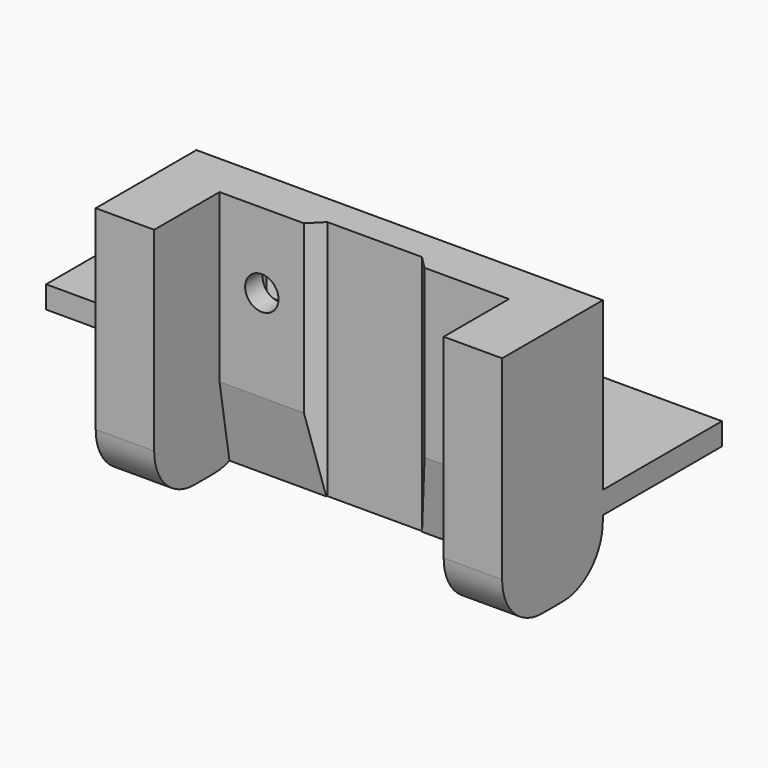
from build123d import *

# Parameters (mm, degrees)
F0_W           = 13.375
F0_H           = 2
F1_DEPTH       = 25
F2_R           = 1.75
F3_DEPTH       = 2
F4_W           = 11.3
F4_H           = 7
F5_DEPTH       = 25
F5_DEPTH_BACK  = 11.5
F6_W           = 26
F6_H           = 6.5
F7_DEPTH       = 7
F9_DEPTH       = 7
F11_DEPTH      = 19.75
F11_DEPTH_BACK = 6.25
F12_T1_DEPTH   = 27.75
F12_T3_DEPTH   = 27.75
F12_T5_DEPTH   = 59
F14_DEPTH      = 15
F15_W          = 5.5
F15_H          = 5.5
F16_DEPTH      = 2
F17_DEPTH      = 2
F18_D          = 3


# Not quite as in the source:
# - a fillet or chamfer that OpenCascade refuses, or shapes differently, is made with other operations: its cross-section is extruded or revolved along the edge and cut away or added


with BuildPart() as f1:
    # F0 (on Right) → F1 (new body, symmetric)
    with BuildSketch(Plane.YZ):
        with Locations((6.6875, 1)):
            Rectangle(F0_W, F0_H)
    extrude(amount=F1_DEPTH, both=True)

    # F2 (on face) → F3 (cut, through all)
    with BuildSketch(Plane.XY.offset(2)):
        with Locations((-13, 4)):
            Circle(F2_R)
        with Locations((13, 4)):
            Circle(F2_R)
    extrude(amount=-F3_DEPTH, mode=Mode.SUBTRACT)

    # F4 (on Right) → F5 (join, two sides)
    with BuildSketch(Plane.YZ) as f5_sk:
        with Locations((-5.65, -1.5)):
            Rectangle(F4_W, F4_H)
    extrude(amount=F5_DEPTH)
    extrude(f5_sk.sketch, amount=-F5_DEPTH_BACK)

    # F6 (on face) → F7 (cut, through all)
    with BuildSketch(Plane(origin=(0, 0, -5), x_dir=(1, 0, 0), z_dir=(0, 0, -1))):
        with Locations((6.75, 8.05)):
            Rectangle(F6_W, F6_H)
    extrude(amount=-F7_DEPTH, mode=Mode.SUBTRACT)

    # F8 (on face) → F9 (cut, through all)
    with BuildSketch(Plane(origin=(0, 0, -5), x_dir=(1, 0, 0), z_dir=(0, 0, -1))):
        Polygon((13, 4.8), (0.5, 4.8), (2.5, 2.8), (11, 2.8), align=None)
    extrude(amount=-F9_DEPTH, mode=Mode.SUBTRACT)

    # F10 (on Right) → F11 (cut, two sides)
    with BuildSketch(Plane.YZ) as f11_sk:
        Polygon((-4.8, -5), (-2.8, -5), (-4.8, 7), align=None)
    extrude(amount=F11_DEPTH, mode=Mode.SUBTRACT)
    extrude(f11_sk.sketch, amount=-F11_DEPTH_BACK, mode=Mode.SUBTRACT)

    # F12: fillet of radius 4.5 on 3 edges, made by hand

    # F12_s2 → F12_t1 (cut)
    with BuildSketch(Plane.YZ.offset(-22.75)):
        with BuildLine():
            ThreePointArc((-6.8, -5), (-9.9819805153, -3.6819805153), (-11.3, -0.5))
            Line((-11.3, -0.5), (-11.3, -5))
            Line((-11.3, -5), (-6.8, -5))
        make_face()
    extrude(amount=F12_T1_DEPTH, mode=Mode.SUBTRACT)

    # F12_s4 → F12_t3 (cut)
    with BuildSketch(Plane.YZ.offset(8.5)):
        with BuildLine():
            ThreePointArc((-6.8, -5), (-9.9819805153, -3.6819805153), (-11.3, -0.5))
            Line((-11.3, -0.5), (-11.3, -5))
            Line((-11.3, -5), (-6.8, -5))
        make_face()
    extrude(amount=F12_T3_DEPTH, mode=Mode.SUBTRACT)

    # F12_s6 → F12_t5 (cut)
    with BuildSketch(Plane.YZ.offset(-22.75)):
        with BuildLine():
            ThreePointArc((0, -0.5), (-1.3180194847, -3.6819805153), (-4.5, -5))
            Line((-4.5, -5), (0, -5))
            Line((0, -5), (0, -0.5))
        make_face()
    extrude(amount=F12_T5_DEPTH, mode=Mode.SUBTRACT)

    # F13 (on face) → F14 (join)
    with BuildSketch(Plane.XY.offset(2)):
        Polygon((25, 0), (-11.5, 0), (-11.5, -11.3), (-6.25, -11.3), (-6.25, -3.9666666667), (1.3333333333, -3.9666666667), (2.5, -2.8), (11, -2.8), (12.1666666667, -3.9666666667), (19.75, -3.9666666667), (19.75, -11.3), (25, -11.3), align=None)
    extrude(amount=F14_DEPTH)

    # F15 (on face) → F16 (join)
    with BuildSketch(Plane(origin=(0, 0, 0), x_dir=(-1, 0, 0), z_dir=(0, 1, 0))):
        with Locations((-16.04918, 10.25)):
            Rectangle(F15_W, F15_H)
        with Locations((2.45082, 10.25)):
            Rectangle(F15_W, F15_H)
    extrude(amount=-F16_DEPTH)

    # F15 (on face) → F17 (cut)
    with BuildSketch(Plane(origin=(0, 0, 0), x_dir=(-1, 0, 0), z_dir=(0, 1, 0))):
        with Locations((-16.04918, 10.25)):
            Rectangle(F15_W, F15_H)
        with Locations((2.45082, 10.25)):
            Rectangle(F15_W, F15_H)
    extrude(amount=-F17_DEPTH, mode=Mode.SUBTRACT)

    # F18 (through all)
    with Locations(Plane(origin=(0, 0, 0), x_dir=(-1, 0, 0), z_dir=(0, 1, 0))):
        with Locations((2.45082, 10.25), (-16.04918, 10.25)):
            Hole(F18_D / 2)


solid = f1.part
